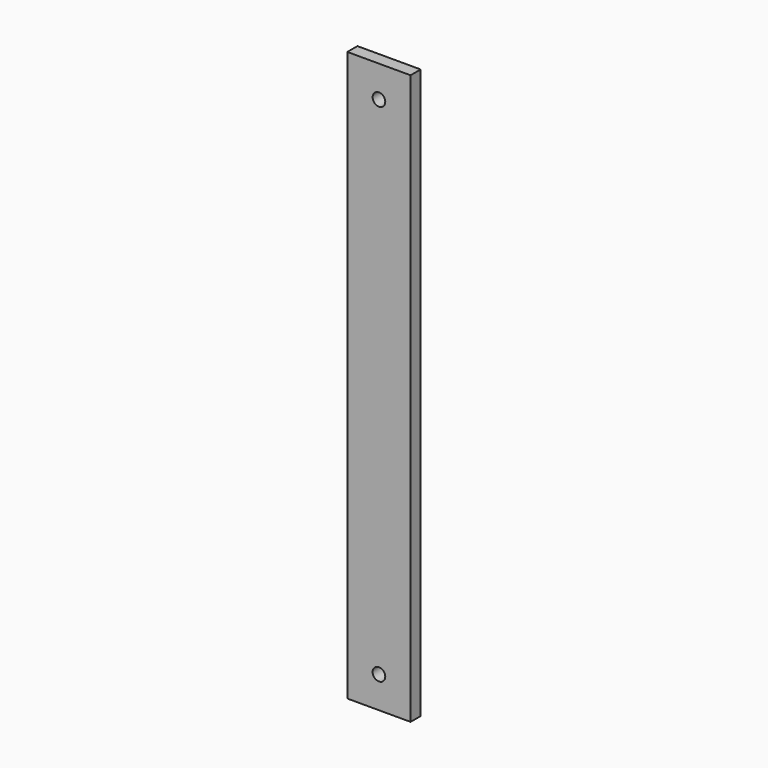
from build123d import *

# Parameters (mm, degrees)
F0_W     = 100
F0_H     = 900
F1_DEPTH = 20
F2_R     = 10
F3_DEPTH = 25


# Not quite as in the source:
# - a pattern or mirror of a feature is missing from the dataset's text; its kind, count and spacing are read off the source's solid


with BuildPart() as f1:
    # F0 (on Front) → F1 (new body)
    with BuildSketch(Plane.XZ):
        Rectangle(F0_W, F0_H)
    extrude(amount=F1_DEPTH)

    # F2 (on face) → F3 (cut)
    with BuildSketch(Plane.XZ.offset(20)):
        with Locations((0, -400)):
            Circle(F2_R)
    f3 = extrude(amount=-F3_DEPTH, mode=Mode.SUBTRACT)

    # F3_copies: F3 across plane
    add(f3.mirror(Plane.XY), mode=Mode.SUBTRACT)


solid = f1.part
